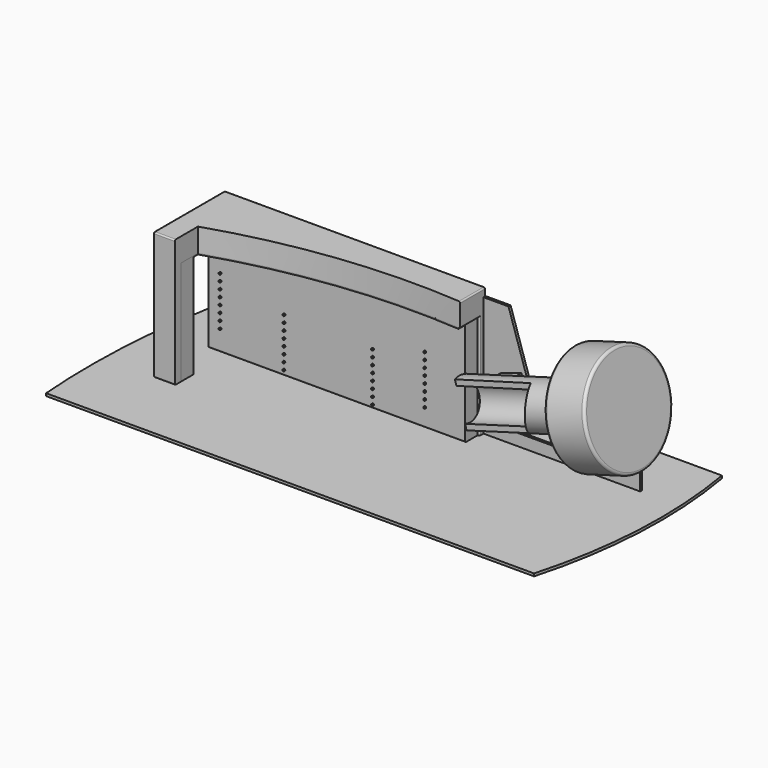
from build123d import *

# Parameters (mm, degrees)
F1_DEPTH      = 496.5
F1_DEPTH_BACK = 3.5
F3_DEPTH      = 493
F5_DEPTH      = 245.091
F5_DEPTH_BACK = 865
F6_R          = 2
F7_DEPTH      = 2
F8_R          = 2.5
F8_2_R        = 2.5
F10_DEPTH     = 5
F15_DEPTH     = 41.1940478204
F17_DEPTH     = 245.091
F19_DEPTH     = 5


# Not quite as in the source:
# - an extrude ends at something that could not be found from the text; its depth is read off the source's solid


with BuildPart() as f1:
    # F0 (on Right) → F1 (new body, two sides)
    with BuildSketch(Plane.YZ) as f1_sk:
        Polygon((0, 245.09), (-171.18, 245.09), (-171.18, 0), (-156.59, 0), (-156.59, 200), (-14.59, 200), (-14.59, 0), (0, 0), align=None)
    extrude(amount=F1_DEPTH)
    extrude(f1_sk.sketch, amount=-F1_DEPTH_BACK)


with BuildPart() as f3:
    # F2 (on Right) → F3 (new body)
    with BuildSketch(Plane.YZ):
        Polygon((-44.59, 0), (-14.59, 0), (-14.59, 200), (-156.59, 200), (-156.59, 0), (-126.59, 0), (-126.59, 198), (-44.59, 198), align=None)
    extrude(amount=F3_DEPTH)


with BuildPart() as f5_tool:
    # F4 (on face) → F5 (new body, two sides)
    with BuildSketch(Plane.XY.offset(245.09)) as f5_sk:
        with BuildLine():
            ThreePointArc((496.5, -60.8477942775), (264.4550156346, -65.7022987418), (37.799552083, -115.659698844))
            Line((37.799552083, -115.659698844), (37.799552083, -171.18))
            Line((37.799552083, -171.18), (496.5, -171.18))
            Line((496.5, -171.18), (496.5, -60.8477942775))
        make_face()
    extrude(amount=-F5_DEPTH)
    extrude(f5_sk.sketch, amount=F5_DEPTH_BACK)


with BuildPart() as f1_1:
    add(f1.part)

    # F5: cut by f5_tool
    add(f5_tool.part, mode=Mode.SUBTRACT)

    # F8
    f8_edges = [f1_1.edges().sort_by_distance(p)[0] for p in [
        (17.149776, -171.18, 245.09),
        (-3.5, -85.59, 245.09),
        (246.5, 0, 245.09),
        (-3.5, -171.18, 122.545),
        (496.5, 0, 122.545),
        (496.5, -30.423897, 245.09),
        (496.5, -14.59, 100),
        (496.5, -37.718897, 200),
        (246.5, 0, 0),
        (-3.5, 0, 122.545),
        (-3.5, -14.59, 100),
        (-3.5, -85.59, 200),
        (-3.5, -156.59, 100),
        (-3.5, -163.885, 0),
        (17.149776, -171.18, 0),
        (-3.5, -7.295, 0),
    ]]
    fillet(f8_edges, radius=F8_R)


with BuildPart() as f3_1:
    add(f3.part)

    # F5: cut by f5_tool
    add(f5_tool.part, mode=Mode.SUBTRACT)

    # F8#2
    f8_2_edges = [f3_1.edges().sort_by_distance(p)[0] for p in [
        (0, -44.59, 99),
        (246.5, -44.59, 0),
    ]]
    fillet(f8_2_edges, radius=F8_2_R)


with BuildPart() as f7:
    # F6 (on face) → F7 (new body)
    with BuildSketch(Plane.XZ.offset(44.59)):
        with Locations((24, 39.75)):
            Circle(F6_R)
    extrude(amount=F7_DEPTH)


with BuildPart() as f7b:
    # F6 (on face) → F7, piece 2 (new body)
    with BuildSketch(Plane.XZ.offset(44.59)):
        with Locations((24, 53.09)):
            Circle(F6_R)
    extrude(amount=F7_DEPTH)


with BuildPart() as f7c:
    # F6 (on face) → F7, piece 3 (new body)
    with BuildSketch(Plane.XZ.offset(44.59)):
        with Locations((24, 66.43)):
            Circle(F6_R)
    extrude(amount=F7_DEPTH)


with BuildPart() as f7d:
    # F6 (on face) → F7, piece 4 (new body)
    with BuildSketch(Plane.XZ.offset(44.59)):
        with Locations((24, 79.77)):
            Circle(F6_R)
    extrude(amount=F7_DEPTH)


with BuildPart() as f7e:
    # F6 (on face) → F7, piece 5 (new body)
    with BuildSketch(Plane.XZ.offset(44.59)):
        with Locations((24, 93.11)):
            Circle(F6_R)
    extrude(amount=F7_DEPTH)


with BuildPart() as f7f:
    # F6 (on face) → F7, piece 6 (new body)
    with BuildSketch(Plane.XZ.offset(44.59)):
        with Locations((24, 106.45)):
            Circle(F6_R)
    extrude(amount=F7_DEPTH)


with BuildPart() as f7g:
    # F6 (on face) → F7, piece 7 (new body)
    with BuildSketch(Plane.XZ.offset(44.59)):
        with Locations((24, 119.79)):
            Circle(F6_R)
    extrude(amount=F7_DEPTH)


with BuildPart() as f7h:
    # F6 (on face) → F7, piece 8 (new body)
    with BuildSketch(Plane.XZ.offset(44.59)):
        with Locations((24, 133.13)):
            Circle(F6_R)
    extrude(amount=F7_DEPTH)


with BuildPart() as f7i:
    # F6 (on face) → F7, piece 9 (new body)
    with BuildSketch(Plane.XZ.offset(44.59)):
        with Locations((146.3, 9.75)):
            Circle(F6_R)
    extrude(amount=F7_DEPTH)


with BuildPart() as f7j:
    # F6 (on face) → F7, piece 10 (new body)
    with BuildSketch(Plane.XZ.offset(44.59)):
        with Locations((146.3530413302, 23.0898945505)):
            Circle(F6_R)
    extrude(amount=F7_DEPTH)


with BuildPart() as f7k:
    # F6 (on face) → F7, piece 11 (new body)
    with BuildSketch(Plane.XZ.offset(44.59)):
        with Locations((146.4060826604, 36.4297891009)):
            Circle(F6_R)
    extrude(amount=F7_DEPTH)


with BuildPart() as f7l:
    # F6 (on face) → F7, piece 12 (new body)
    with BuildSketch(Plane.XZ.offset(44.59)):
        with Locations((146.4591239907, 49.7696836514)):
            Circle(F6_R)
    extrude(amount=F7_DEPTH)


with BuildPart() as f7m:
    # F6 (on face) → F7, piece 13 (new body)
    with BuildSketch(Plane.XZ.offset(44.59)):
        with Locations((146.5121653209, 63.1095782018)):
            Circle(F6_R)
    extrude(amount=F7_DEPTH)


with BuildPart() as f7n:
    # F6 (on face) → F7, piece 14 (new body)
    with BuildSketch(Plane.XZ.offset(44.59)):
        with Locations((146.5652066511, 76.4494727523)):
            Circle(F6_R)
    extrude(amount=F7_DEPTH)


with BuildPart() as f7o:
    # F6 (on face) → F7, piece 15 (new body)
    with BuildSketch(Plane.XZ.offset(44.59)):
        with Locations((146.6182479813, 89.7893673027)):
            Circle(F6_R)
    extrude(amount=F7_DEPTH)


with BuildPart() as f7p:
    # F6 (on face) → F7, piece 16 (new body)
    with BuildSketch(Plane.XZ.offset(44.59)):
        with Locations((146.6712893115, 103.1292618532)):
            Circle(F6_R)
    extrude(amount=F7_DEPTH)


with BuildPart() as f7q:
    # F6 (on face) → F7, piece 17 (new body)
    with BuildSketch(Plane.XZ.offset(44.59)):
        with Locations((316.3, 6.75)):
            Circle(F6_R)
    extrude(amount=F7_DEPTH)


with BuildPart() as f7r:
    # F6 (on face) → F7, piece 18 (new body)
    with BuildSketch(Plane.XZ.offset(44.59)):
        with Locations((316.3, 20.09)):
            Circle(F6_R)
    extrude(amount=F7_DEPTH)


with BuildPart() as f7s:
    # F6 (on face) → F7, piece 19 (new body)
    with BuildSketch(Plane.XZ.offset(44.59)):
        with Locations((316.3, 33.43)):
            Circle(F6_R)
    extrude(amount=F7_DEPTH)


with BuildPart() as f7t:
    # F6 (on face) → F7, piece 20 (new body)
    with BuildSketch(Plane.XZ.offset(44.59)):
        with Locations((316.3, 46.77)):
            Circle(F6_R)
    extrude(amount=F7_DEPTH)


with BuildPart() as f7u:
    # F6 (on face) → F7, piece 21 (new body)
    with BuildSketch(Plane.XZ.offset(44.59)):
        with Locations((316.3, 60.11)):
            Circle(F6_R)
    extrude(amount=F7_DEPTH)


with BuildPart() as f7v:
    # F6 (on face) → F7, piece 22 (new body)
    with BuildSketch(Plane.XZ.offset(44.59)):
        with Locations((316.3, 73.45)):
            Circle(F6_R)
    extrude(amount=F7_DEPTH)


with BuildPart() as f7w:
    # F6 (on face) → F7, piece 23 (new body)
    with BuildSketch(Plane.XZ.offset(44.59)):
        with Locations((316.3, 86.79)):
            Circle(F6_R)
    extrude(amount=F7_DEPTH)


with BuildPart() as f7x:
    # F6 (on face) → F7, piece 24 (new body)
    with BuildSketch(Plane.XZ.offset(44.59)):
        with Locations((316.3, 100.13)):
            Circle(F6_R)
    extrude(amount=F7_DEPTH)


with BuildPart() as f7y:
    # F6 (on face) → F7, piece 25 (new body)
    with BuildSketch(Plane.XZ.offset(44.59)):
        with Locations((416.3, 34.75)):
            Circle(F6_R)
    extrude(amount=F7_DEPTH)


with BuildPart() as f7z:
    # F6 (on face) → F7, piece 26 (new body)
    with BuildSketch(Plane.XZ.offset(44.59)):
        with Locations((416.3, 48.09)):
            Circle(F6_R)
    extrude(amount=F7_DEPTH)


with BuildPart() as f7ba:
    # F6 (on face) → F7, piece 27 (new body)
    with BuildSketch(Plane.XZ.offset(44.59)):
        with Locations((416.3, 61.43)):
            Circle(F6_R)
    extrude(amount=F7_DEPTH)


with BuildPart() as f7bb:
    # F6 (on face) → F7, piece 28 (new body)
    with BuildSketch(Plane.XZ.offset(44.59)):
        with Locations((416.3, 74.77)):
            Circle(F6_R)
    extrude(amount=F7_DEPTH)


with BuildPart() as f7bc:
    # F6 (on face) → F7, piece 29 (new body)
    with BuildSketch(Plane.XZ.offset(44.59)):
        with Locations((416.3, 88.11)):
            Circle(F6_R)
    extrude(amount=F7_DEPTH)


with BuildPart() as f7bd:
    # F6 (on face) → F7, piece 30 (new body)
    with BuildSketch(Plane.XZ.offset(44.59)):
        with Locations((416.3, 101.45)):
            Circle(F6_R)
    extrude(amount=F7_DEPTH)


with BuildPart() as f7be:
    # F6 (on face) → F7, piece 31 (new body)
    with BuildSketch(Plane.XZ.offset(44.59)):
        with Locations((416.3, 114.79)):
            Circle(F6_R)
    extrude(amount=F7_DEPTH)


with BuildPart() as f7bf:
    # F6 (on face) → F7, piece 32 (new body)
    with BuildSketch(Plane.XZ.offset(44.59)):
        with Locations((416.3, 128.13)):
            Circle(F6_R)
    extrude(amount=F7_DEPTH)


with BuildPart() as f10:
    # F9 (on Front) → F10 (new body)
    with BuildSketch(Plane.XZ):
        Polygon((496.5, 230), (496.5, 0), (796.5, 0), (796.5, 90), (589.81, 90), (544.38, 230), align=None)
        with BuildLine():
            ThreePointArc((544, 55), (547.6611652352, 63.8388347648), (556.5, 67.5))
            Line((556.5, 67.5), (736.5, 67.5))
            ThreePointArc((736.5, 67.5), (745.3388347648, 63.8388347648), (749, 55))
            Line((749, 55), (749, 35))
            ThreePointArc((749, 35), (745.3388347648, 26.1611652352), (736.5, 22.5))
            Line((736.5, 22.5), (556.5, 22.5))
            ThreePointArc((556.5, 22.5), (547.6611652352, 26.1611652352), (544, 35))
            Line((544, 35), (544, 55))
        make_face(mode=Mode.SUBTRACT)
    extrude(amount=F10_DEPTH)



with BuildPart() as f13:
    # F12 (on offset) → F13 (revolve)
    with BuildSketch(Plane.XZ.offset(85)):
        with BuildLine():
            Line((765.7995671735, 163.9935185238), (838.3567513404, 184.7989562873))
            Line((838.3567513404, 184.7989562873), (812.1712025378, 276.1188174015))
            ThreePointArc((812.1712025378, 276.1188174015), (809.7889421594, 279.1137291581), (805.986707279, 279.5469391021))
            Line((805.986707279, 279.5469391021), (738.6983885634, 260.2523241949))
            ThreePointArc((738.6983885634, 260.2523241949), (735.7034768067, 257.8700638164), (735.2702668627, 254.0678289361))
            Line((735.2702668627, 254.0678289361), (748.3630412641, 208.407898379))
            ThreePointArc((748.3630412641, 208.407898379), (747.9298313201, 204.6056634987), (744.9349195634, 202.2234031203))
            Line((744.9349195634, 202.2234031203), (514.2321125382, 136.0704377242))
            Line((514.2321125382, 136.0704377242), (516.9884860964, 126.4578207648))
            Line((516.9884860964, 126.4578207648), (756.8413531094, 195.2345236418))
            Line((756.8413531094, 195.2345236418), (765.7995671735, 163.9935185238))
        make_face()
    revolve(axis=Axis((708.5270167557, -85, 147.5708789609), (0.9612616959, 0, 0.2756373558)))


with BuildPart() as f10_1:
    add(f10.part)

    add(f13.part)  # F15 merges F13
    # F14 (on face) → F15 (join, through all)
    with BuildSketch(Plane.XZ.offset(5)):
        Polygon((568.9997785028, 125.5910519579), (529.200626934, 112.6762272738), (532.3213916163, 103.0590787919), (572.1205431851, 115.973903476), align=None)
    extrude(amount=F15_DEPTH)

    # F16 (on face) → F17 (cut, through all)
    with BuildSketch(Plane.XY.offset(245.09)):
        Polygon((660.9079173015, -97.4862553808), (497.634857893, -96.1695387959), (497.1029758453, -162.1229946613), (688.0488991737, -162.1229946613), align=None)
    extrude(amount=-F17_DEPTH, mode=Mode.SUBTRACT)


with BuildPart() as f19:
    # F18 (on face) → F19 (new body)
    with BuildSketch(Plane(origin=(0, 0, 0), x_dir=(1, 0, 0), z_dir=(0, 0, -1))):
        with BuildLine():
            Line((838.5716676712, 311.5820586681), (-96.478164196, 311.5820586681))
            ThreePointArc((-96.478164196, 311.5820586681), (-97.3530672768, 98.7834409447), (-66.6927322745, -111.7966175079))
            Line((-66.6927322745, -111.7966175079), (859.847009182, -111.7966175079))
            ThreePointArc((859.847009182, -111.7966175079), (872.8452335678, 101.0804557433), (838.5716676712, 311.5820586681))
        make_face()
        with BuildLine():
            Line((-1, 14.59), (494, 14.59))
            ThreePointArc((494, 14.59), (495.767766953, 13.857766953), (496.5, 12.09))
            Line((496.5, 12.09), (496.5, 2.5))
            Line((496.5, 2.5), (-1, 2.5))
            Line((-1, 2.5), (-1, 14.59))
        make_face(mode=Mode.SUBTRACT)
    extrude(amount=F19_DEPTH)


solid = Compound([f1_1.part, f3_1.part, f7.part, f7b.part, f7c.part, f7d.part, f7e.part, f7f.part, f7g.part, f7h.part, f7i.part, f7j.part, f7k.part, f7l.part, f7m.part, f7n.part, f7o.part, f7p.part, f7q.part, f7r.part, f7s.part, f7t.part, f7u.part, f7v.part, f7w.part, f7x.part, f7y.part, f7z.part, f7ba.part, f7bb.part, f7bc.part, f7bd.part, f7be.part, f7bf.part, f10_1.part, f19.part])
